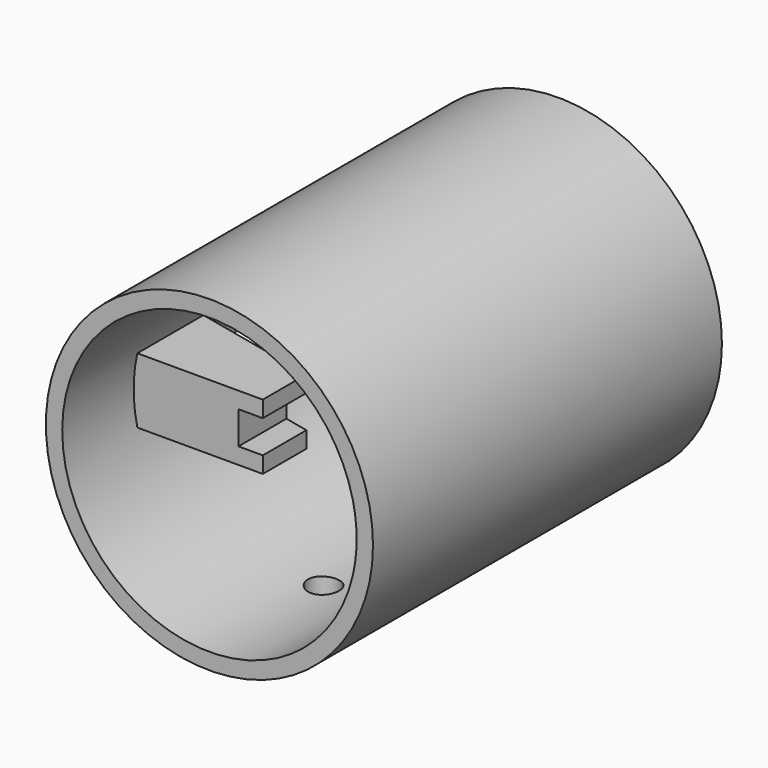
from build123d import *

# Parameters (mm, degrees)
F0_R      = 30
F1_DEPTH  = 80
F2_R      = 27.5
F3_DEPTH  = 2
F4_W      = 13.5446311965
F4_H      = 18
F5_DEPTH  = 6
F6_R      = 2.851632841
F7_DEPTH  = 34.4
F9_DEPTH  = 6
F8_W      = 24
F8_H      = 10
F10_DEPTH = 6
F11_W     = 5.1813843587
F11_H     = 18
F12_DEPTH = 3
F13_DEPTH = 60
F15_DEPTH = 50


# Not quite as in the source:
# - a feature names something its author has since deleted; it is built from what else it names


with BuildPart() as f1:
    # F0 (on Front) → F1 (new body)
    with BuildSketch(Plane.XZ):
        Circle(F0_R)
        with BuildLine():
            ThreePointArc((26.3248931622, 6), (26.8306924564, 3.0189306568), (27, 0))
            ThreePointArc((27, 0), (26.8306924564, -3.0189306568), (26.3248931622, -6))
            ThreePointArc((26.3248931622, -6), (-27, 0), (26.3248931622, 6))
        make_face(mode=Mode.SUBTRACT)
    extrude(amount=F1_DEPTH)

    # F4 (on Top) → F5 (cut, symmetric)
    with BuildSketch(Plane.XY):
        with Locations((-25.5865128711, -31.3380542621)):
            Rectangle(F4_W, F4_H)
    extrude(amount=F5_DEPTH, both=True, mode=Mode.SUBTRACT)

    # F6 (on Top) → F7 (cut)
    with BuildSketch(Plane.XY):
        with Locations((0, -53.8231134415)):
            Circle(F6_R)
    extrude(amount=-F7_DEPTH, mode=Mode.SUBTRACT)

    # F8 (on Top) → F9 (join, symmetric)
    with BuildSketch(Plane.XY):
        Polygon((-27.3131299764, -53.6233463883), (-3.3131299764, -53.6233463883), (-27.464909479, -48.2202917337), align=None)
    extrude(amount=F9_DEPTH, both=True)

    # F8 (on Top) → F10 (join, symmetric)
    with BuildSketch(Plane.XY):
        with Locations((-15.3131299764, -58.6233463883)):
            Rectangle(F8_W, F8_H)
    extrude(amount=F10_DEPTH, both=True)

    # F11 (on Top) → F12 (cut, symmetric)
    with BuildSketch(Plane.XY):
        with Locations((-5.1839929656, -58.0122377723)):
            Rectangle(F11_W, F11_H)
    extrude(amount=F12_DEPTH, both=True, mode=Mode.SUBTRACT)

    # F14 (on Right) → F15 (cut)
    with BuildSketch(Plane.YZ):
        with BuildLine():
            add(Edge.make_bspline(
                [(-15.5778108165, -5.2500003949), (-8.3745810525, -5.2500003949), (-11.9761959345, 2.6250001974), (-15.5778108165, 10.5000007898), (-19.1794256985, 2.6250001974), (-22.7810405805, -5.2500003949), (-15.5778108165, -5.2500003949)],
                knots=[0, 0, 0, 2.0943951024, 2.0943951024, 4.1887902048, 4.1887902048, 6.2831853072, 6.2831853072, 6.2831853072], degree=2, weights=[1, 0.5, 1, 0.5, 1, 0.5, 1]))
        make_face()
    extrude(amount=-F15_DEPTH, mode=Mode.SUBTRACT)


with BuildPart() as f3:
    # F2 (on Front) → F3 (new body)
    with BuildSketch(Plane.XZ):
        with Locations((-0.0819229608, 0.1413219288)):
            Circle(F2_R)
    extrude(amount=F3_DEPTH)


with BuildPart() as f13:
    # F0 (on Front) → F13 (new body)
    with BuildSketch(Plane.XZ):
        with BuildLine():
            Line((24.1553578526, 0), (27, 0))
            ThreePointArc((27, 0), (26.8306924564, 3.0189306568), (26.3248931622, 6))
            Line((26.3248931622, 6), (17, 6))
            Line((17, 6), (17, 1.6203357372))
            Line((17, 1.6203357372), (24.1553578526, 1.6203357372))
            Line((24.1553578526, 1.6203357372), (24.1553578526, 0))
        make_face()
        with BuildLine():
            ThreePointArc((26.3248931622, -6), (26.8306924564, -3.0189306568), (27, 0))
            Line((27, 0), (24.1553578526, 0))
            Line((24.1553578526, 0), (24.1553578526, -1.6203357372))
            Line((24.1553578526, -1.6203357372), (17, -1.6203357372))
            Line((17, -1.6203357372), (17, -6))
            Line((17, -6), (26.3248931622, -6))
        make_face()
    extrude(amount=F13_DEPTH)


solid = Compound([f1.part, f3.part, f13.part])
